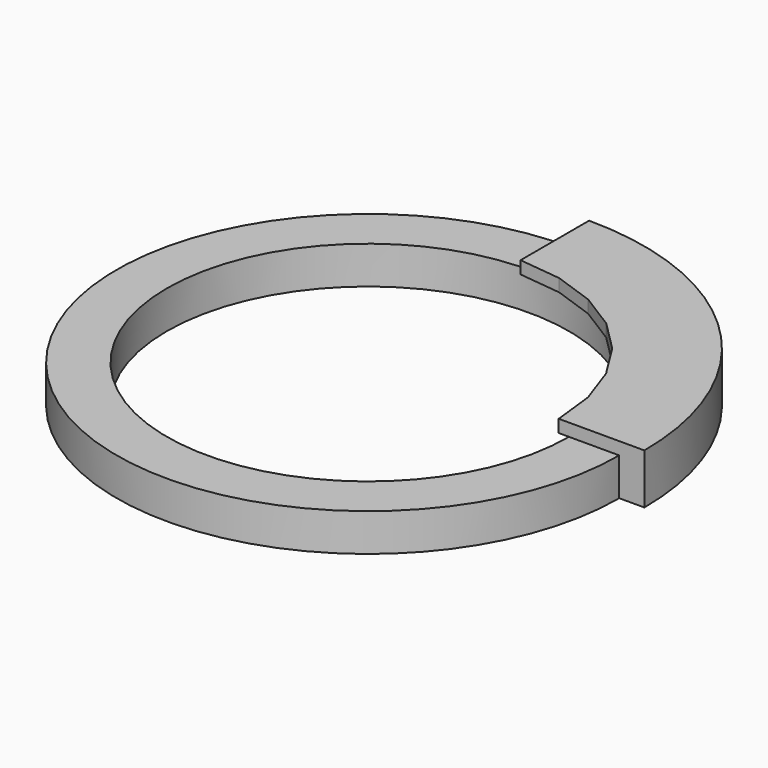
from build123d import *

# Parameters (mm, degrees)
F0_R     = 50.8
F1_DEPTH = 9.525
F2_R     = 63.5
F3_DEPTH = 9.525
F6_DEPTH = 9.525
F7_DEPTH = 3.175
F9_DEPTH = 25.4


# Not quite as in the source:
# - a length typed as a fraction of an inch, garbled in the dataset ("3 / 203.2 mm" for 3/8 in), is restored


with BuildPart() as f1:
    # F0 (on Top) → F1 (new body)
    with BuildSketch(Plane.XY):
        Circle(F0_R)
    extrude(amount=F1_DEPTH)


with BuildPart() as f3:
    # F2 (on Top) → F3 (new body)
    with BuildSketch(Plane.XY):
        Circle(F2_R)
    extrude(amount=F3_DEPTH)

    # F4: cut F1
    add(f1.part, mode=Mode.SUBTRACT)


with BuildPart() as f6:
    # F5 (on face) → F6 (new body)
    with BuildSketch(Plane.XY.offset(9.525)):
        with BuildLine():
            Line((63.5, 0), (69.85, 0))
            ThreePointArc((69.85, 0), (49.3914086659, 49.3914086659), (0, 69.85))
            Line((0, 69.85), (0, 63.5))
            ThreePointArc((0, 63.5), (44.9012806053, 44.9012806053), (63.5, 0))
        make_face()
    extrude(amount=-F6_DEPTH)

    # F5 (on face) → F7 (join)
    with BuildSketch(Plane.XY.offset(9.525)):
        with BuildLine():
            Line((63.5, 0), (69.85, 0))
            ThreePointArc((69.85, 0), (49.3914086659, 49.3914086659), (0, 69.85))
            Line((0, 69.85), (0, 63.5))
            ThreePointArc((0, 63.5), (44.9012806053, 44.9012806053), (63.5, 0))
        make_face()
        with BuildLine():
            Line((30.1279164851, 0), (63.5, 0))
            ThreePointArc((63.5, 0), (44.9012806053, 44.9012806053), (0, 63.5))
            Line((0, 63.5), (0, 30.1279164851))
            ThreePointArc((0, 30.1279164851), (21.3036540496, 21.3036540496), (30.1279164851, 0))
        make_face()
    extrude(amount=F7_DEPTH)

    # F8 (on face) → F9 (cut)
    with BuildSketch(Plane.XY.offset(12.7)):
        Polygon((47.0000967019, -10.7274653679), (48.2087917626, 0), (47.0000967019, 10.7274653679), (43.4346205373, 20.9170108283), (37.6911511317, 30.0576900239), (30.0576900239, 37.6911511317), (20.9170108283, 43.4346205373), (10.7274653679, 47.0000967019), (0, 48.2087917626), (-10.7274653679, 47.0000967019), (-20.9170108283, 43.4346205373), (-30.0576900239, 37.6911511317), (-37.6911511317, 30.0576900239), (-43.4346205373, 20.9170108283), (-47.0000967019, 10.7274653679), (-48.2087917626, 0), (-47.0000967019, -10.7274653679), (-43.4346205373, -20.9170108283), (-37.6911511317, -30.0576900239), (-30.0576900239, -37.6911511317), (-20.9170108283, -43.4346205373), (-10.7274653679, -47.0000967019), (0, -48.2087917626), (10.7274653679, -47.0000967019), (20.9170108283, -43.4346205373), (30.0576900239, -37.6911511317), (37.6911511317, -30.0576900239), (43.4346205373, -20.9170108283), align=None)
    extrude(amount=-F9_DEPTH, mode=Mode.SUBTRACT)


solid = Compound([f3.part, f6.part])
